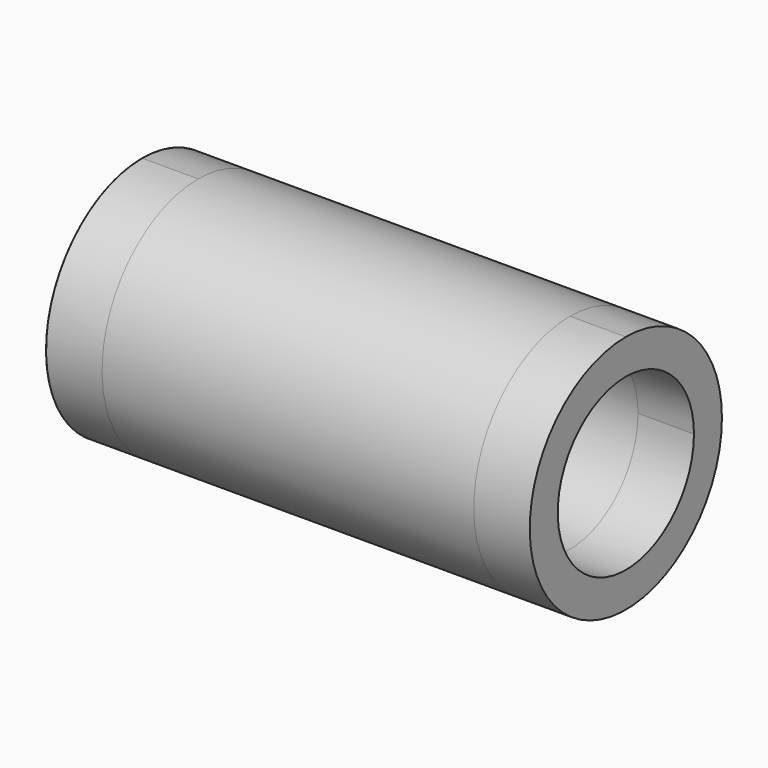
from build123d import *

# Parameters (mm, degrees)
F1_W     = 17.6168819889
F1_H     = 11.0105499625
F5_R     = 37.8028899431
F5_R_2   = 26.7923399806
F6_DEPTH = 152.2524452932


# Not quite as in the source:
# - a pattern or mirror of a feature is missing from the dataset's text; its kind, count and spacing are read off the source's solid
# - the program builds the solid bodies; features that only make, move or delete a surface that nothing else refers to are left out


with BuildPart() as f2:
    # F1 (on Front) → F2 (revolve)
    with BuildSketch(Plane.XZ):
        with Locations((13.7020186521, 32.2976149619)):
            Rectangle(F1_W, F1_H)
    revolve(axis=Axis((44.2868806422, 0, 0), (1, 0, 0)))


with BuildPart() as f2_copies_1:
    # F2_copies: instance of F2
    add(f2.part.mirror(Plane(origin=(-53.615263, 0, 0), x_dir=(0, 0, -1), z_dir=(-1, 0, 0))))


with BuildPart() as f2_1:
    add(f2.part)

    add(f2_copies_1.part)  # F6 merges F2_copies_1
    # F5 (on face) → F6 (join, through all)
    with BuildSketch(Plane.YZ.offset(22.5104596466)):
        Circle(F5_R)
        Circle(F5_R_2, mode=Mode.SUBTRACT)
    extrude(amount=-F6_DEPTH)


solid = f2_1.part
